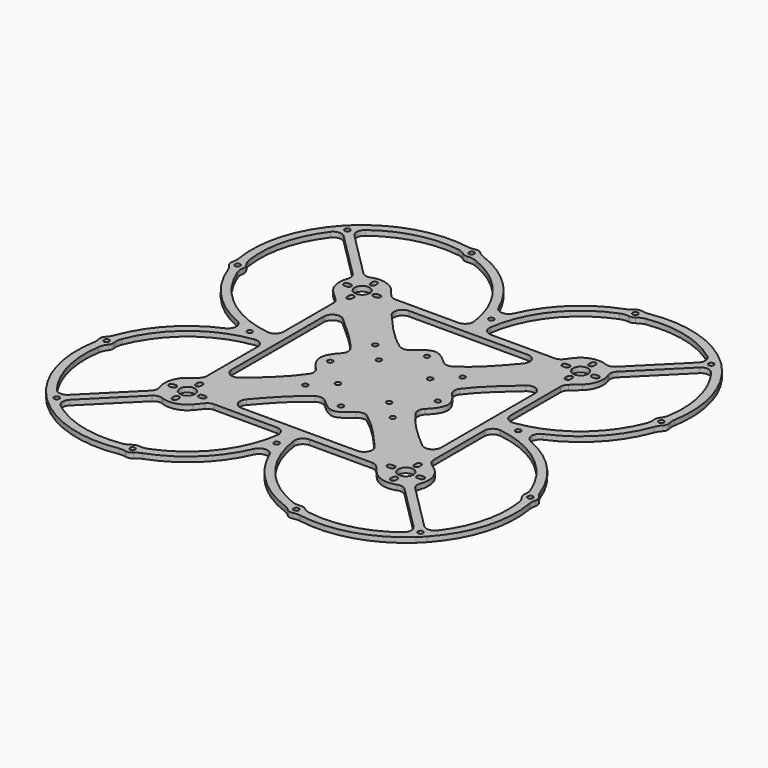
from build123d import *

# Parameters (mm, degrees)
F0_R     = 1.55
F0_R_2   = 4.5
F1_DEPTH = 3


# Not quite as in the source:
# - a feature names something its author has since deleted; it is built from what else it names


with BuildPart() as f1:
    # F0 (on Top) → F1 (new body)
    with BuildSketch(Plane.XY):
        with BuildLine():
            ThreePointArc((4.5936412885, 90.9640892891), (1.5876e-06, 87.9385448385), (-4.5936380583, 90.9640893729))
            ThreePointArc((-4.5936380583, 90.9640893729), (-19.7997665524, 112.7493601662), (-42.3857157583, 126.7386155355))
            ThreePointArc((-42.3857157583, 126.7386155355), (-44.282976849, 127.6715883742), (-45.9416856044, 128.9825892242))
            ThreePointArc((-45.9416856044, 128.9825892242), (-47.711537449, 129.9897804476), (-49.7479021723, 129.9951119953))
            ThreePointArc((-49.7479021723, 129.9951119953), (-51.8387697531, 129.6815665856), (-53.9488258268, 129.814612931))
            ThreePointArc((-53.9488258268, 129.814612931), (-83.7536549239, 128.0187505985), (-109.6908840175, 113.2264179235))
            ThreePointArc((-109.6908840175, 113.2264179235), (-111.492270863, 111.492270863), (-113.2264179235, 109.6908840175))
            ThreePointArc((-113.2264179235, 109.6908840175), (-128.0187505985, 83.7536549239), (-129.814612931, 53.9488258268))
            ThreePointArc((-129.814612931, 53.9488258268), (-129.6815665856, 51.8387697531), (-129.9951119953, 49.7479021723))
            ThreePointArc((-129.9951119953, 49.7479021723), (-129.9897804476, 47.711537449), (-128.9825892242, 45.9416856044))
            ThreePointArc((-128.9825892242, 45.9416856044), (-127.6715883742, 44.282976849), (-126.7386155355, 42.3857157583))
            ThreePointArc((-126.7386155355, 42.3857157583), (-112.7493601662, 19.7997665524), (-90.9640893729, 4.5936380583))
            ThreePointArc((-90.9640893729, 4.5936380583), (-87.9385448385, -1.5876e-06), (-90.9640892891, -4.5936412885))
            ThreePointArc((-90.9640892891, -4.5936412885), (-112.7493564136, -19.7997669532), (-126.7386107311, -42.3857113668))
            ThreePointArc((-126.7386107311, -42.3857113668), (-127.6715848934, -44.2829742089), (-128.9825877652, -45.9416841141))
            ThreePointArc((-128.9825877652, -45.9416841141), (-129.9897804476, -47.711537449), (-129.9951114697, -49.7479041907))
            ThreePointArc((-129.9951114697, -49.7479041907), (-129.6815648767, -51.8387737737), (-129.8146109437, -53.9488320249))
            ThreePointArc((-129.8146109437, -53.9488320249), (-128.0187466409, -83.7536577022), (-113.2264144939, -109.6908833036))
            ThreePointArc((-113.2264144939, -109.6908833036), (-111.4922673823, -111.4922701), (-109.6908804846, -113.2264171062))
            ThreePointArc((-109.6908804846, -113.2264171062), (-83.7536558603, -128.018747189), (-53.9488320249, -129.8146109437))
            ThreePointArc((-53.9488320249, -129.8146109437), (-51.8387737737, -129.6815648767), (-49.7479041907, -129.9951114697))
            ThreePointArc((-49.7479041907, -129.9951114697), (-47.711537449, -129.9897804476), (-45.9416841141, -128.9825877652))
            ThreePointArc((-45.9416841141, -128.9825877652), (-44.2829742089, -127.6715848934), (-42.3857113668, -126.7386107311))
            ThreePointArc((-42.3857113668, -126.7386107311), (-19.7997655576, -112.7493550925), (-4.5936397708, -90.9640857581))
            ThreePointArc((-4.5936397708, -90.9640857581), (0, -87.938541039), (4.5936397708, -90.9640857581))
            ThreePointArc((4.5936397708, -90.9640857581), (19.7997655576, -112.7493550925), (42.3857113668, -126.7386107311))
            ThreePointArc((42.3857113668, -126.7386107311), (44.2829742089, -127.6715848934), (45.9416841141, -128.9825877652))
            ThreePointArc((45.9416841141, -128.9825877652), (47.711537449, -129.9897804476), (49.7479041907, -129.9951114697))
            ThreePointArc((49.7479041907, -129.9951114697), (51.8387737737, -129.6815648767), (53.9488320249, -129.8146109437))
            ThreePointArc((53.9488320249, -129.8146109437), (83.7536567813, -128.0187469149), (109.6908818941, -113.2264158001))
            ThreePointArc((109.6908818941, -113.2264158001), (111.4922687411, -111.4922687411), (113.2264158001, -109.6908818941))
            ThreePointArc((113.2264158001, -109.6908818941), (128.0187469149, -83.7536567813), (129.8146109437, -53.9488320249))
            ThreePointArc((129.8146109437, -53.9488320249), (129.6815648767, -51.8387737737), (129.9951114697, -49.7479041907))
            ThreePointArc((129.9951114697, -49.7479041907), (129.9897804476, -47.711537449), (128.9825877652, -45.9416841141))
            ThreePointArc((128.9825877652, -45.9416841141), (127.6715848934, -44.2829742089), (126.7386107311, -42.3857113668))
            ThreePointArc((126.7386107311, -42.3857113668), (112.7493550925, -19.7997655576), (90.9640857581, -4.5936397708))
            ThreePointArc((90.9640857581, -4.5936397708), (87.938541039, 0), (90.9640857581, 4.5936397708))
            ThreePointArc((90.9640857581, 4.5936397708), (112.7493550925, 19.7997655576), (126.7386107311, 42.3857113668))
            ThreePointArc((126.7386107311, 42.3857113668), (127.6715848934, 44.2829742089), (128.9825877652, 45.9416841141))
            ThreePointArc((128.9825877652, 45.9416841141), (129.9897804476, 47.711537449), (129.9951114697, 49.7479041907))
            ThreePointArc((129.9951114697, 49.7479041907), (129.6815648767, 51.8387737737), (129.8146109437, 53.9488320249))
            ThreePointArc((129.8146109437, 53.9488320249), (128.018747189, 83.7536558603), (113.2264171062, 109.6908804846))
            ThreePointArc((113.2264171062, 109.6908804846), (111.4922701, 111.4922673823), (109.6908833036, 113.2264144939))
            ThreePointArc((109.6908833036, 113.2264144939), (83.7536577022, 128.0187466408), (53.9488320249, 129.8146109437))
            ThreePointArc((53.9488320249, 129.8146109437), (51.8387737737, 129.6815648767), (49.7479041907, 129.9951114697))
            ThreePointArc((49.7479041907, 129.9951114697), (47.711537449, 129.9897804476), (45.9416841141, 128.9825877652))
            ThreePointArc((45.9416841141, 128.9825877652), (44.2829742089, 127.6715848934), (42.3857113668, 126.7386107311))
            ThreePointArc((42.3857113668, 126.7386107311), (19.7997669532, 112.7493564136), (4.5936412885, 90.9640892891))
        make_face()
        with Locations((-108.2905437355, -108.153230011)):
            Circle(F0_R, mode=Mode.SUBTRACT)
        with Locations((-48.7398474892, -126.1242172983)):
            Circle(F0_R, mode=Mode.SUBTRACT)
        with BuildLine():
            Line((-66.5, -74.5), (-66.5, -73))
            ThreePointArc((-66.5, -73), (-65, -71.5), (-63.5, -73))
            Line((-63.5, -73), (-63.5, -74.5))
            ThreePointArc((-63.5, -74.5), (-65, -76), (-66.5, -74.5))
        make_face(mode=Mode.SUBTRACT)
        with Locations((-126.1242172983, -48.7398474892)):
            Circle(F0_R, mode=Mode.SUBTRACT)
        with BuildLine():
            Line((-73, -66.5), (-74.5, -66.5))
            ThreePointArc((-74.5, -66.5), (-76, -65), (-74.5, -63.5))
            Line((-74.5, -63.5), (-73, -63.5))
            ThreePointArc((-73, -63.5), (-71.5, -65), (-73, -66.5))
        make_face(mode=Mode.SUBTRACT)
        with Locations((-79.8885448385, 0)):
            Circle(F0_R, mode=Mode.SUBTRACT)
        with Locations((-65, -65)):
            Circle(F0_R_2, mode=Mode.SUBTRACT)
        with BuildLine():
            ThreePointArc((-57, -66.5), (-58.5, -65), (-57, -63.5))
            Line((-57, -63.5), (-55.5, -63.5))
            ThreePointArc((-55.5, -63.5), (-54, -65), (-55.5, -66.5))
            Line((-55.5, -66.5), (-57, -66.5))
        make_face(mode=Mode.SUBTRACT)
        with BuildLine():
            Line((-66.5, -57), (-66.5, -55.5))
            ThreePointArc((-66.5, -55.5), (-65, -54), (-63.5, -55.5))
            Line((-63.5, -55.5), (-63.5, -57))
            ThreePointArc((-63.5, -57), (-65, -58.5), (-66.5, -57))
        make_face(mode=Mode.SUBTRACT)
        with Locations((48.7398474892, -126.1242172983)):
            Circle(F0_R, mode=Mode.SUBTRACT)
        with Locations((0, -79.8885448385)):
            Circle(F0_R, mode=Mode.SUBTRACT)
        with BuildLine():
            ThreePointArc((66.5, -74.5), (65, -76), (63.5, -74.5))
            Line((63.5, -74.5), (63.5, -73))
            ThreePointArc((63.5, -73), (65, -71.5), (66.5, -73))
            Line((66.5, -73), (66.5, -74.5))
        make_face(mode=Mode.SUBTRACT)
        with Locations((108.2784277556, -108.1560280507)):
            Circle(F0_R, mode=Mode.SUBTRACT)
        with BuildLine():
            ThreePointArc((57, -63.5), (58.5, -65), (57, -66.5))
            Line((57, -66.5), (55.5, -66.5))
            ThreePointArc((55.5, -66.5), (54, -65), (55.5, -63.5))
            Line((55.5, -63.5), (57, -63.5))
        make_face(mode=Mode.SUBTRACT)
        with Locations((65, -65)):
            Circle(F0_R_2, mode=Mode.SUBTRACT)
        with BuildLine():
            ThreePointArc((66.5, -57), (65, -58.5), (63.5, -57))
            Line((63.5, -57), (63.5, -55.5))
            ThreePointArc((63.5, -55.5), (65, -54), (66.5, -55.5))
            Line((66.5, -55.5), (66.5, -57))
        make_face(mode=Mode.SUBTRACT)
        with BuildLine():
            ThreePointArc((-78.7260276961, 75.1904937901), (-77.3700677078, 72.6909557736), (-77.5962746825, 69.8563220777))
            ThreePointArc((-77.5962746825, 69.8563220777), (-78.1774623607, 62.066659629), (-74.3468847944, 55.2590685948))
            ThreePointArc((-74.3468847944, 55.2590685948), (-55.8574100489, 55.0670724866), (-54.5192604238, 73.5090597562))
            ThreePointArc((-54.5192604238, 73.5090597562), (-61.5236729853, 78.0447365051), (-69.8563220777, 77.5962746825))
            ThreePointArc((-69.8563220777, 77.5962746825), (-72.6909557736, 77.3700677078), (-75.1904937901, 78.7260276961))
            Line((-75.1904937901, 78.7260276961), (-102.2950830455, 105.8306169514))
            ThreePointArc((-102.2950830455, 105.8306169514), (-103.7481732445, 109.7032406669), (-101.7873113942, 113.3451778401))
            ThreePointArc((-101.7873113942, 113.3451778401), (-80.0827992563, 123.8478688365), (-56.0022199647, 125.0799671641))
            ThreePointArc((-56.0022199647, 125.0799671641), (-53.4825995412, 124.3550905641), (-51.2379870694, 123.0002296802))
            ThreePointArc((-51.2379870694, 123.0002296802), (-49.7681575294, 122.258654149), (-48.1241365653, 122.1718888632))
            ThreePointArc((-48.1241365653, 122.1718888632), (-45.5030157293, 122.2323762703), (-42.9562600942, 121.6095047758))
            ThreePointArc((-42.9562600942, 121.6095047758), (-17.2773803845, 102.5914096175), (-4.8022395632, 73.1726457399))
            ThreePointArc((-4.8022395632, 73.1726457399), (-5.9909393236, 69.2108685569), (-9.7567877473, 67.5))
            Line((-9.7567877473, 67.5), (-47.2749619701, 67.5))
            ThreePointArc((-47.2749619701, 67.5), (-49.4332948043, 67.989833775), (-51.1687379105, 69.3633602493))
            add(Edge.make_bspline(
                [(-51.1687379105, 69.3633602493), (-47.007111135, 64.1971813129), (-42.9204896878, 59.0857782526), (-38.8861434054, 54.2837422746)],
                knots=[0.0293673697, 0.0293673697, 0.0293673697, 0.0293673697, 0.1393383892, 0.1393383892, 0.1393383892, 0.1393383892], degree=3))
            ThreePointArc((-38.8861434054, 54.2837422746), (-39.5900475875, 59.6117186571), (-35.0578688274, 62.5))
            Line((-35.0578688274, 62.5), (35.6142056633, 62.5))
            ThreePointArc((35.6142056633, 62.5), (40.1396288907, 59.6261572409), (39.4629102085, 54.3082178452))
            add(Edge.make_bspline(
                [(39.4629102085, 54.3082178452), (43.4572386204, 59.1246461501), (47.4477718972, 64.2594353508), (51.4265936274, 69.4628891406)],
                knots=[0.8640600007, 0.8640600007, 0.8640600007, 0.8640600007, 0.9739367654, 0.9739367654, 0.9739367654, 0.9739367654], degree=3))
            ThreePointArc((51.4265936274, 69.4628891406), (49.6699228907, 68.0175032461), (47.4546976535, 67.5))
            Line((47.4546976535, 67.5), (9.7567877473, 67.5))
            ThreePointArc((9.7567877473, 67.5), (5.9909393236, 69.2108685569), (4.8022395632, 73.1726457399))
            ThreePointArc((4.8022395632, 73.1726457399), (17.2773803845, 102.5914096175), (42.9562600942, 121.6095047758))
            ThreePointArc((42.9562600942, 121.6095047758), (45.5030157293, 122.2323762703), (48.1241365653, 122.1718888632))
            ThreePointArc((48.1241365653, 122.1718888632), (49.7681575294, 122.258654149), (51.2379870694, 123.0002296802))
            ThreePointArc((51.2379870694, 123.0002296802), (53.4825995412, 124.3550905641), (56.0022199647, 125.0799671641))
            ThreePointArc((56.0022199647, 125.0799671641), (80.0828001163, 123.8478686161), (101.7873128072, 113.3451767649))
            ThreePointArc((101.7873128072, 113.3451767649), (103.748174551, 109.7032395344), (102.2950842388, 105.8306158614))
            Line((102.2950842388, 105.8306158614), (75.1904941913, 78.7260273982))
            ThreePointArc((75.1904941913, 78.7260273982), (72.6909561352, 77.370067483), (69.8563224458, 77.5962745406))
            ThreePointArc((69.8563224458, 77.5962745406), (61.3181994895, 77.9882387182), (54.2558912586, 73.1739909073))
            ThreePointArc((54.2558912586, 73.1739909073), (55.8750675797, 55.0508488641), (74.0703287451, 55.0010432317))
            ThreePointArc((74.0703287451, 55.0010432317), (78.1350771686, 61.8823489971), (77.5962748245, 69.8563217095))
            ThreePointArc((77.5962748245, 69.8563217095), (77.3700679326, 72.6909554121), (78.7260279939, 75.190493389))
            Line((78.7260279939, 75.190493389), (105.8306180414, 102.2950818521))
            ThreePointArc((105.8306180414, 102.2950818521), (109.7032417994, 103.7481719379), (113.3451789152, 101.7873099812))
            ThreePointArc((113.3451789152, 101.7873099812), (123.8478690569, 80.0827983963), (125.0799671641, 56.0022199647))
            ThreePointArc((125.0799671641, 56.0022199647), (124.3550905641, 53.4825995412), (123.0002296802, 51.2379870694))
            ThreePointArc((123.0002296802, 51.2379870694), (122.258654149, 49.7681575294), (122.1718888632, 48.1241365653))
            ThreePointArc((122.1718888632, 48.1241365653), (122.2323762703, 45.5030157293), (121.6095047758, 42.9562600942))
            ThreePointArc((121.6095047758, 42.9562600942), (102.5914096175, 17.2773803845), (73.1726457399, 4.8022395632))
            ThreePointArc((73.1726457399, 4.8022395632), (69.2108685569, 5.9909393236), (67.5, 9.7567877473))
            Line((67.5, 9.7567877473), (67.5, 46.9024650002))
            ThreePointArc((67.5, 46.9024650002), (67.9450696625, 48.9646506418), (69.2010438482, 50.6597097764))
            add(Edge.make_bspline(
                [(69.2010438482, 50.6597097764), (64.0951140729, 46.1765740091), (59.0182901872, 41.9052788751), (54.2353248312, 37.7820833857)],
                knots=[0.0348728398, 0.0348728398, 0.0348728398, 0.0348728398, 0.1445829675, 0.1445829675, 0.1445829675, 0.1445829675], degree=3))
            ThreePointArc((54.2353248312, 37.7820833857), (59.5828615119, 38.5405267444), (62.5, 33.9950138006))
            Line((62.5, 33.9950138006), (62.5, -35.5495988309))
            ThreePointArc((62.5, -35.5495988309), (59.6206264771, -40.0776164264), (54.2988226622, -39.3904924316))
            add(Edge.make_bspline(
                [(54.2988226622, -39.3904924316), (59.1121784473, -43.4021644694), (64.2467475497, -47.4153572737), (69.4560669959, -51.4128712838)],
                knots=[0.8650150287, 0.8650150287, 0.8650150287, 0.8650150287, 0.9740421792, 0.9740421792, 0.9740421792, 0.9740421792], degree=3))
            ThreePointArc((69.4560669959, -51.4128712838), (68.0156012097, -49.6575734697), (67.5, -47.4462011605))
            Line((67.5, -47.4462011605), (67.5, -9.7567877473))
            ThreePointArc((67.5, -9.7567877473), (69.2108685569, -5.9909393236), (73.1726457399, -4.8022395632))
            ThreePointArc((73.1726457399, -4.8022395632), (102.5914096175, -17.2773803845), (121.6095047758, -42.9562600942))
            ThreePointArc((121.6095047758, -42.9562600942), (122.2323762703, -45.5030157293), (122.1718888632, -48.1241365653))
            ThreePointArc((122.1718888632, -48.1241365653), (122.258654149, -49.7681575294), (123.0002296802, -51.2379870694))
            ThreePointArc((123.0002296802, -51.2379870694), (124.3550905641, -53.4825995412), (125.0799671641, -56.0022199647))
            ThreePointArc((125.0799671641, -56.0022199647), (123.8478688365, -80.0827992563), (113.3451778401, -101.7873113942))
            ThreePointArc((113.3451778401, -101.7873113942), (109.7032406669, -103.7481732445), (105.8306169514, -102.2950830455))
            Line((105.8306169514, -102.2950830455), (78.7260276961, -75.1904937901))
            ThreePointArc((78.7260276961, -75.1904937901), (77.3700677078, -72.6909557736), (77.5962746825, -69.8563220777))
            ThreePointArc((77.5962746825, -69.8563220777), (77.9903375994, -61.3256117442), (73.1862480092, -54.2652273647))
            ThreePointArc((73.1862480092, -54.2652273647), (55.0961710642, -55.8258966427), (54.9219208197, -73.9823337745))
            ThreePointArc((54.9219208197, -73.9823337745), (61.8248103944, -78.1212869403), (69.8563220777, -77.5962746825))
            ThreePointArc((69.8563220777, -77.5962746825), (72.6909557736, -77.3700677078), (75.1904937901, -78.7260276961))
            Line((75.1904937901, -78.7260276961), (102.2950830455, -105.8306169514))
            ThreePointArc((102.2950830455, -105.8306169514), (103.7481732445, -109.7032406669), (101.7873113942, -113.3451778401))
            ThreePointArc((101.7873113942, -113.3451778401), (80.0827992563, -123.8478688365), (56.0022199647, -125.0799671641))
            ThreePointArc((56.0022199647, -125.0799671641), (53.4825995412, -124.3550905641), (51.2379870694, -123.0002296802))
            ThreePointArc((51.2379870694, -123.0002296802), (49.7681575294, -122.258654149), (48.1241365653, -122.1718888632))
            ThreePointArc((48.1241365653, -122.1718888632), (45.5030157293, -122.2323762703), (42.9562600942, -121.6095047758))
            ThreePointArc((42.9562600942, -121.6095047758), (17.2773803845, -102.5914096175), (4.8022395632, -73.1726457399))
            ThreePointArc((4.8022395632, -73.1726457399), (5.9909393236, -69.2108685569), (9.7567877473, -67.5))
            Line((9.7567877473, -67.5), (46.9610754937, -67.5))
            ThreePointArc((46.9610754937, -67.5), (49.0351777215, -67.9504835478), (50.7355403773, -69.2207600206))
            add(Edge.make_bspline(
                [(50.7355403773, -69.2207600206), (46.2776004608, -64.0895900624), (42.0082462932, -59.0081310929), (37.8793761718, -54.2306155101)],
                knots=[0.0336445481, 0.0336445481, 0.0336445481, 0.0336445481, 0.1425668185, 0.1425668185, 0.1425668185, 0.1425668185], degree=3))
            ThreePointArc((37.8793761718, -54.2306155101), (38.6431792121, -59.5800333592), (34.0963714061, -62.5))
            Line((34.0963714061, -62.5), (-34.6716965747, -62.5))
            ThreePointArc((-34.6716965747, -62.5), (-39.2116462302, -59.594959934), (-38.4761016269, -54.25554285))
            add(Edge.make_bspline(
                [(-38.4761016269, -54.25554285), (-42.5524815665, -59.0354489236), (-46.7247402937, -64.1334390375), (-51.0163929038, -69.3081210856)],
                knots=[0.86152407, 0.86152407, 0.86152407, 0.86152407, 0.9696650908, 0.9696650908, 0.9696650908, 0.9696650908], degree=3))
            ThreePointArc((-51.0163929038, -69.3081210856), (-49.2938689584, -67.974550046), (-47.1677686047, -67.5))
            Line((-47.1677686047, -67.5), (-9.7567877474, -67.5))
            ThreePointArc((-9.7567877474, -67.5), (-5.9909393237, -69.2108685569), (-4.8022395633, -73.1726457399))
            ThreePointArc((-4.8022395633, -73.1726457399), (-17.2773803846, -102.5914096175), (-42.9562600944, -121.6095047758))
            ThreePointArc((-42.9562600944, -121.6095047758), (-45.5030157294, -122.2323762703), (-48.1241365654, -122.1718888632))
            ThreePointArc((-48.1241365654, -122.1718888632), (-49.7681575294, -122.258654149), (-51.2379870693, -123.0002296802))
            ThreePointArc((-51.2379870693, -123.0002296802), (-53.4825995411, -124.355090564), (-56.0022199645, -125.079967164))
            ThreePointArc((-56.0022199645, -125.079967164), (-80.0827983962, -123.8478690568), (-101.7873099811, -113.3451789152))
            ThreePointArc((-101.7873099811, -113.3451789152), (-103.7481719378, -109.7032417994), (-102.295081852, -105.8306180414))
            Line((-102.295081852, -105.8306180414), (-75.190493389, -78.7260279939))
            ThreePointArc((-75.190493389, -78.7260279939), (-72.6909554121, -77.3700679326), (-69.8563217095, -77.5962748245))
            ThreePointArc((-69.8563217095, -77.5962748245), (-61.6280970797, -78.0721180647), (-54.6566830252, -73.6755860873))
            ThreePointArc((-54.6566830252, -73.6755860873), (-55.3115936341, -55.5986818962), (-73.3606290294, -54.4004772639))
            ThreePointArc((-73.3606290294, -54.4004772639), (-78.019936228, -61.431910789), (-77.5962745406, -69.8563224458))
            ThreePointArc((-77.5962745406, -69.8563224458), (-77.370067483, -72.6909561352), (-78.7260273982, -75.1904941913))
            Line((-78.7260273982, -75.1904941913), (-105.8306158613, -102.2950842388))
            ThreePointArc((-105.8306158613, -102.2950842388), (-109.7032395344, -103.7481745509), (-113.3451767648, -101.7873128071))
            ThreePointArc((-113.3451767648, -101.7873128071), (-123.847868616, -80.0828001162), (-125.079967164, -56.0022199645))
            ThreePointArc((-125.079967164, -56.0022199645), (-124.355090564, -53.4825995411), (-123.0002296802, -51.2379870693))
            ThreePointArc((-123.0002296802, -51.2379870693), (-122.258654149, -49.7681575294), (-122.1718888632, -48.1241365654))
            ThreePointArc((-122.1718888632, -48.1241365654), (-122.2323762703, -45.5030157294), (-121.6095047758, -42.9562600944))
            ThreePointArc((-121.6095047758, -42.9562600944), (-102.5915462524, -17.277488013), (-73.1729904451, -4.8022863626))
            ThreePointArc((-73.1729904451, -4.8022863626), (-69.2111956733, -5.9909728541), (-67.5003163344, -9.7568306947))
            Line((-67.5003163344, -9.7568306947), (-67.5003163328, -47.353236691))
            ThreePointArc((-67.5003163328, -47.353236691), (-68.0006204029, -49.5333138774), (-69.4014109482, -51.2771104681))
            add(Edge.make_bspline(
                [(-54.2790618736, -39.0485616103), (-59.0828616964, -43.094423634), (-64.2057413604, -47.1737958924), (-69.4014109482, -51.2771104681)],
                knots=[0.8641405018, 0.8641405018, 0.8641405018, 0.8641405018, 0.9725362801, 0.9725362801, 0.9725362801, 0.9725362801], degree=3))
            ThreePointArc((-54.2790618736, -39.0485616103), (-59.6089463445, -39.7576935316), (-62.5, -35.2242240748))
            Line((-62.5, -35.2242240748), (-62.5, 33.4095018987))
            ThreePointArc((-62.5, 33.4095018987), (-59.5674116994, 37.9620625919), (-54.209676454, 37.1743087945))
            add(Edge.make_bspline(
                [(-69.1233391423, 50.3680202269), (-64.0476785875, 45.7195000527), (-58.9859996351, 41.3486659558), (-54.209676454, 37.1743087945)],
                knots=[0.0376140132, 0.0376140132, 0.0376140132, 0.0376140132, 0.147134592, 0.147134592, 0.147134592, 0.147134592], degree=3))
            ThreePointArc((-69.1233391423, 50.3680202269), (-67.9240249358, 48.6950792761), (-67.5003163367, 46.6807414163))
            Line((-67.5003163367, 46.6807414163), (-67.5003163352, 9.7568306951))
            ThreePointArc((-67.5003163352, 9.7568306951), (-69.211195674, 5.9909728542), (-73.1729904459, 4.8022863626))
            ThreePointArc((-73.1729904459, 4.8022863626), (-102.5915462527, 17.2774880132), (-121.6095047758, 42.9562600942))
            ThreePointArc((-121.6095047758, 42.9562600942), (-122.2323762703, 45.5030157293), (-122.1718888632, 48.1241365653))
            ThreePointArc((-122.1718888632, 48.1241365653), (-122.258654149, 49.7681575294), (-123.0002296802, 51.2379870694))
            ThreePointArc((-123.0002296802, 51.2379870694), (-124.3550905641, 53.4825995412), (-125.0799671641, 56.0022199647))
            ThreePointArc((-125.0799671641, 56.0022199647), (-123.8478688365, 80.0827992563), (-113.3451778401, 101.7873113942))
            ThreePointArc((-113.3451778401, 101.7873113942), (-109.7032406669, 103.7481732445), (-105.8306169514, 102.2950830455))
            Line((-105.8306169514, 102.2950830455), (-78.7260276961, 75.1904937901))
        make_face(mode=Mode.SUBTRACT)
        with BuildLine():
            ThreePointArc((74.5, -63.5), (76, -65), (74.5, -66.5))
            Line((74.5, -66.5), (73, -66.5))
            ThreePointArc((73, -66.5), (71.5, -65), (73, -63.5))
            Line((73, -63.5), (74.5, -63.5))
        make_face(mode=Mode.SUBTRACT)
        with Locations((126.1242172983, -48.7398474892)):
            Circle(F0_R, mode=Mode.SUBTRACT)
        with Locations((79.8885448385, 0)):
            Circle(F0_R, mode=Mode.SUBTRACT)
        with Locations((-126.1242172983, 48.7398474892)):
            Circle(F0_R, mode=Mode.SUBTRACT)
        with BuildLine():
            ThreePointArc((-73, 66.5), (-71.5, 65), (-73, 63.5))
            Line((-73, 63.5), (-74.5, 63.5))
            ThreePointArc((-74.5, 63.5), (-76, 65), (-74.5, 66.5))
            Line((-74.5, 66.5), (-73, 66.5))
        make_face(mode=Mode.SUBTRACT)
        with BuildLine():
            ThreePointArc((-63.5, 55.5), (-65, 54), (-66.5, 55.5))
            Line((-66.5, 55.5), (-66.5, 57))
            ThreePointArc((-66.5, 57), (-65, 58.5), (-63.5, 57))
            Line((-63.5, 57), (-63.5, 55.5))
        make_face(mode=Mode.SUBTRACT)
        with Locations((-65, 65)):
            Circle(F0_R_2, mode=Mode.SUBTRACT)
        with BuildLine():
            Line((-55.5, 63.5), (-57, 63.5))
            ThreePointArc((-57, 63.5), (-58.5, 65), (-57, 66.5))
            Line((-57, 66.5), (-55.5, 66.5))
            ThreePointArc((-55.5, 66.5), (-54, 65), (-55.5, 63.5))
        make_face(mode=Mode.SUBTRACT)
        with Locations((-108.3014905595, 108.1507019099)):
            Circle(F0_R, mode=Mode.SUBTRACT)
        with BuildLine():
            ThreePointArc((-63.5, 73), (-65, 71.5), (-66.5, 73))
            Line((-66.5, 73), (-66.5, 74.5))
            ThreePointArc((-66.5, 74.5), (-65, 76), (-63.5, 74.5))
            Line((-63.5, 74.5), (-63.5, 73))
        make_face(mode=Mode.SUBTRACT)
        with Locations((-48.7398474892, 126.1242172983)):
            Circle(F0_R, mode=Mode.SUBTRACT)
        with BuildLine():
            Line((63.5, 55.5), (63.5, 57))
            ThreePointArc((63.5, 57), (65, 58.5), (66.5, 57))
            Line((66.5, 57), (66.5, 55.5))
            ThreePointArc((66.5, 55.5), (65, 54), (63.5, 55.5))
        make_face(mode=Mode.SUBTRACT)
        with BuildLine():
            Line((55.5, 66.5), (57, 66.5))
            ThreePointArc((57, 66.5), (58.5, 65), (57, 63.5))
            Line((57, 63.5), (55.5, 63.5))
            ThreePointArc((55.5, 63.5), (54, 65), (55.5, 66.5))
        make_face(mode=Mode.SUBTRACT)
        with Locations((65, 65)):
            Circle(F0_R_2, mode=Mode.SUBTRACT)
        with BuildLine():
            Line((74.5, 63.5), (73, 63.5))
            ThreePointArc((73, 63.5), (71.5, 65), (73, 66.5))
            Line((73, 66.5), (74.5, 66.5))
            ThreePointArc((74.5, 66.5), (76, 65), (74.5, 63.5))
        make_face(mode=Mode.SUBTRACT)
        with Locations((126.1242172983, 48.7398474892)):
            Circle(F0_R, mode=Mode.SUBTRACT)
        with Locations((0, 79.8885448385)):
            Circle(F0_R, mode=Mode.SUBTRACT)
        with BuildLine():
            Line((66.5, 74.5), (66.5, 73))
            ThreePointArc((66.5, 73), (65, 71.5), (63.5, 73))
            Line((63.5, 73), (63.5, 74.5))
            ThreePointArc((63.5, 74.5), (65, 76), (66.5, 74.5))
        make_face(mode=Mode.SUBTRACT)
        with Locations((48.7398474892, 126.1242172983)):
            Circle(F0_R, mode=Mode.SUBTRACT)
        with Locations((108.153230011, 108.2905437356)):
            Circle(F0_R, mode=Mode.SUBTRACT)
        with BuildLine():
            ThreePointArc((-54.5192604238, 73.5090597562), (-55.8574100489, 55.0670724866), (-74.3468847944, 55.2590685948))
            add(Edge.make_bspline(
                [(-74.3468847944, 55.2590685948), (-72.6113826473, 53.5937721304), (-70.8665363109, 51.9645192675), (-69.1233391423, 50.3680202269)],
                knots=[0, 0, 0, 0, 0.0376140132, 0.0376140132, 0.0376140132, 0.0376140132], degree=3))
            add(Edge.make_bspline(
                [(-69.1233391423, 50.3680202269), (-64.0476785875, 45.7195000527), (-58.9859996351, 41.3486659558), (-54.209676454, 37.1743087945)],
                knots=[0.0376140132, 0.0376140132, 0.0376140132, 0.0376140132, 0.147134592, 0.147134592, 0.147134592, 0.147134592], degree=3))
            add(Edge.make_bspline(
                [(-54.209676454, 37.1743087945), (-45.5797737114, 29.6320435523), (-37.8814314438, 22.7311886683), (-32.7153317801, 15.99273753)],
                knots=[0.147134592, 0.147134592, 0.147134592, 0.147134592, 0.3450173373, 0.3450173373, 0.3450173373, 0.3450173373], degree=3))
            add(Edge.make_bspline(
                [(-32.7153317801, 15.99273753), (-31.7544055806, 14.7393443196), (-30.8810906196, 13.4915699994), (-30.1056880744, 12.2463319262)],
                knots=[0.3450173373, 0.3450173373, 0.3450173373, 0.3450173373, 0.3818247408, 0.3818247408, 0.3818247408, 0.3818247408], degree=3))
            add(Edge.make_bspline(
                [(-30.1056880744, 12.2463319262), (-27.5692779158, 8.1730482903), (-24.5965263706, 0.0936378541), (-27.2387091268, -8.3077722195), (-29.6226546248, -12.5690364936)],
                knots=[0.3818247408, 0.3818247408, 0.3818247408, 0.3818247408, 0.5022250058, 0.622241972, 0.622241972, 0.622241972, 0.622241972], degree=3))
            add(Edge.make_bspline(
                [(-29.6226546248, -12.5690364936), (-30.3158734916, -13.8081540799), (-31.099141907, -15.0529586505), (-31.9642401019, -16.3031308824)],
                knots=[0.622241972, 0.622241972, 0.622241972, 0.622241972, 0.6571412704, 0.6571412704, 0.6571412704, 0.6571412704], degree=3))
            add(Edge.make_bspline(
                [(-31.9642401019, -16.3031308824), (-37.0954223742, -23.718314074), (-45.105430893, -31.3223351702), (-54.2790618736, -39.0485616103)],
                knots=[0.6571412704, 0.6571412704, 0.6571412704, 0.6571412704, 0.8641405018, 0.8641405018, 0.8641405018, 0.8641405018], degree=3))
            add(Edge.make_bspline(
                [(-54.2790618736, -39.0485616103), (-59.0828616964, -43.094423634), (-64.2057413604, -47.1737958924), (-69.4014109482, -51.2771104681)],
                knots=[0.8641405018, 0.8641405018, 0.8641405018, 0.8641405018, 0.9725362801, 0.9725362801, 0.9725362801, 0.9725362801], degree=3))
            add(Edge.make_bspline(
                [(-69.4014109482, -51.2771104681), (-70.7178128987, -52.3167476543), (-72.0388875207, -53.3579217921), (-73.3606290294, -54.4004772639)],
                knots=[0.9725362801, 0.9725362801, 0.9725362801, 0.9725362801, 1, 1, 1, 1], degree=3))
            ThreePointArc((-73.3606290294, -54.4004772639), (-55.3115936341, -55.5986818962), (-54.6566830252, -73.6755860873))
            add(Edge.make_bspline(
                [(-51.0163929038, -69.3081210856), (-52.2202551514, -70.7596841376), (-53.4335121775, -72.2172818685), (-54.6566830252, -73.6755860873)],
                knots=[0.9696650908, 0.9696650908, 0.9696650908, 0.9696650908, 1, 1, 1, 1], degree=3))
            add(Edge.make_bspline(
                [(-38.4761016269, -54.25554285), (-42.5524815665, -59.0354489236), (-46.7247402937, -64.1334390375), (-51.0163929038, -69.3081210856)],
                knots=[0.86152407, 0.86152407, 0.86152407, 0.86152407, 0.9696650908, 0.9696650908, 0.9696650908, 0.9696650908], degree=3))
            add(Edge.make_bspline(
                [(-15.7360450393, -31.8416919699), (-23.0709377017, -36.9605236646), (-30.5942962957, -45.0134482139), (-38.4761016269, -54.25554285)],
                knots=[0.6524300978, 0.6524300978, 0.6524300978, 0.6524300978, 0.86152407, 0.86152407, 0.86152407, 0.86152407], degree=3))
            add(Edge.make_bspline(
                [(-12.477120742, -29.7592614372), (-13.5596368679, -30.3847557024), (-14.6457588788, -31.0808094851), (-15.7360450393, -31.8416919699)],
                knots=[0.6213495797, 0.6213495797, 0.6213495797, 0.6213495797, 0.6524300978, 0.6524300978, 0.6524300978, 0.6524300978], degree=3))
            add(Edge.make_bspline(
                [(12.3175276915, -29.9149197418), (8.1902094221, -27.4521418277), (0.0009395531, -24.6081106332), (-8.2746234397, -27.3309946433), (-12.477120742, -29.7592614372)],
                knots=[0.3806340257, 0.3806340257, 0.3806340257, 0.3806340257, 0.500690136, 0.6213495797, 0.6213495797, 0.6213495797, 0.6213495797], degree=3))
            add(Edge.make_bspline(
                [(15.5878401798, -32.071279466), (14.4939747649, -31.2842343393), (13.4042625324, -30.5633762915), (12.3175276915, -29.9149197418)],
                knots=[0.3490229046, 0.3490229046, 0.3490229046, 0.3490229046, 0.3806340257, 0.3806340257, 0.3806340257, 0.3806340257], degree=3))
            add(Edge.make_bspline(
                [(37.8793761718, -54.2306155101), (30.0533332369, -45.1751012959), (22.7320085602, -37.2115671391), (15.5878401798, -32.071279466)],
                knots=[0.1425668185, 0.1425668185, 0.1425668185, 0.1425668185, 0.3490229046, 0.3490229046, 0.3490229046, 0.3490229046], degree=3))
            add(Edge.make_bspline(
                [(50.7355403773, -69.2207600206), (46.2776004608, -64.0895900624), (42.0082462932, -59.0081310929), (37.8793761718, -54.2306155101)],
                knots=[0.0336445481, 0.0336445481, 0.0336445481, 0.0336445481, 0.1425668185, 0.1425668185, 0.1425668185, 0.1425668185], degree=3))
            add(Edge.make_bspline(
                [(54.9219208197, -73.9823337745), (53.5075225493, -72.3953945536), (52.112534936, -70.8057058127), (50.7355403773, -69.2207600206)],
                knots=[0, 0, 0, 0, 0.0336445481, 0.0336445481, 0.0336445481, 0.0336445481], degree=3))
            ThreePointArc((54.9219208197, -73.9823337745), (55.0961710642, -55.8258966427), (73.1862480092, -54.2652273647))
            add(Edge.make_bspline(
                [(69.4560669959, -51.4128712838), (70.6963321973, -52.3646227688), (71.940834612, -53.3154855034), (73.1862480092, -54.2652273647)],
                knots=[0.9740421792, 0.9740421792, 0.9740421792, 0.9740421792, 1, 1, 1, 1], degree=3))
            add(Edge.make_bspline(
                [(54.2988226622, -39.3904924316), (59.1121784473, -43.4021644694), (64.2467475497, -47.4153572737), (69.4560669959, -51.4128712838)],
                knots=[0.8650150287, 0.8650150287, 0.8650150287, 0.8650150287, 0.9740421792, 0.9740421792, 0.9740421792, 0.9740421792], degree=3))
            add(Edge.make_bspline(
                [(31.7459765479, -16.2369208779), (36.8685062051, -23.8659236611), (44.9819221427, -31.6253591313), (54.2988226622, -39.3904924316)],
                knots=[0.6539782468, 0.6539782468, 0.6539782468, 0.6539782468, 0.8650150287, 0.8650150287, 0.8650150287, 0.8650150287], degree=3))
            add(Edge.make_bspline(
                [(29.5219284636, -12.5813755873), (30.1816388577, -13.7962022099), (30.9254369782, -15.0148881949), (31.7459765479, -16.2369208779)],
                knots=[0.620173849, 0.620173849, 0.620173849, 0.620173849, 0.6539782468, 0.6539782468, 0.6539782468, 0.6539782468], degree=3))
            add(Edge.make_bspline(
                [(29.9400645414, 12.3562593878), (27.4904286095, 8.253307767), (24.6482914319, 0.0993554776), (27.2148947835, -8.3330782148), (29.5219284636, -12.5813755873)],
                knots=[0.3828924385, 0.3828924385, 0.3828924385, 0.3828924385, 0.5019585155, 0.620173849, 0.620173849, 0.620173849, 0.620173849], degree=3))
            add(Edge.make_bspline(
                [(32.387471575, 16.0209488062), (31.487130896, 14.7969542017), (30.668363937, 13.5761048132), (29.9400645414, 12.3562593878)],
                knots=[0.3474929937, 0.3474929937, 0.3474929937, 0.3474929937, 0.3828924385, 0.3828924385, 0.3828924385, 0.3828924385], degree=3))
            add(Edge.make_bspline(
                [(54.2353248312, 37.7820833857), (45.3891804875, 30.1561902961), (37.5482347411, 23.0369000102), (32.387471575, 16.0209488062)],
                knots=[0.1445829675, 0.1445829675, 0.1445829675, 0.1445829675, 0.3474929937, 0.3474929937, 0.3474929937, 0.3474929937], degree=3))
            add(Edge.make_bspline(
                [(69.2010438482, 50.6597097764), (64.0951140729, 46.1765740091), (59.0182901872, 41.9052788751), (54.2353248312, 37.7820833857)],
                knots=[0.0348728398, 0.0348728398, 0.0348728398, 0.0348728398, 0.1445829675, 0.1445829675, 0.1445829675, 0.1445829675], degree=3))
            add(Edge.make_bspline(
                [(74.0703287451, 55.0010432317), (72.4499615375, 53.5311635631), (70.8240323045, 52.0847347804), (69.2010438482, 50.6597097764)],
                knots=[0, 0, 0, 0, 0.0348728398, 0.0348728398, 0.0348728398, 0.0348728398], degree=3))
            ThreePointArc((74.0703287451, 55.0010432317), (55.8750675797, 55.0508488641), (54.2558912586, 73.1739909073))
            add(Edge.make_bspline(
                [(51.4265936274, 69.4628891406), (52.3703870168, 70.6971704484), (53.3135214459, 71.9353152278), (54.2558912586, 73.1739909073)],
                knots=[0.9739367654, 0.9739367654, 0.9739367654, 0.9739367654, 1, 1, 1, 1], degree=3))
            add(Edge.make_bspline(
                [(39.4629102085, 54.3082178452), (43.4572386204, 59.1246461501), (47.4477718972, 64.2594353508), (51.4265936274, 69.4628891406)],
                knots=[0.8640600007, 0.8640600007, 0.8640600007, 0.8640600007, 0.9739367654, 0.9739367654, 0.9739367654, 0.9739367654], degree=3))
            add(Edge.make_bspline(
                [(16.0277732624, 31.5601593801), (23.8144639959, 36.6758763345), (31.6459546013, 44.8824014468), (39.4629102085, 54.3082178452)],
                knots=[0.6490296618, 0.6490296618, 0.6490296618, 0.6490296618, 0.8640600007, 0.8640600007, 0.8640600007, 0.8640600007], degree=3))
            add(Edge.make_bspline(
                [(12.63212765, 29.5293297846), (13.7629393959, 30.1370057165), (14.8948821775, 30.8158701398), (16.0277732624, 31.5601593801)],
                knots=[0.6177447473, 0.6177447473, 0.6177447473, 0.6177447473, 0.6490296618, 0.6490296618, 0.6490296618, 0.6490296618], degree=3))
            add(Edge.make_bspline(
                [(-12.5423950306, 29.6621706825), (-8.3687174631, 27.3442678436), (-0.0340331605, 24.699772843), (8.4024067679, 27.2563611954), (12.63212765, 29.5293297846)],
                knots=[0.3834666456, 0.3834666456, 0.3834666456, 0.3834666456, 0.5007257504, 0.6177447473, 0.6177447473, 0.6177447473, 0.6177447473], degree=3))
            add(Edge.make_bspline(
                [(-15.948348592, 31.7675257886), (-14.8125086537, 30.9963498788), (-13.6773755118, 30.292495962), (-12.5423950306, 29.6621706825)],
                knots=[0.3515794687, 0.3515794687, 0.3515794687, 0.3515794687, 0.3834666456, 0.3834666456, 0.3834666456, 0.3834666456], degree=3))
            add(Edge.make_bspline(
                [(-38.8861434054, 54.2837422746), (-31.0999647029, 45.0159433197), (-23.5085002785, 36.9004733616), (-15.948348592, 31.7675257886)],
                knots=[0.1393383892, 0.1393383892, 0.1393383892, 0.1393383892, 0.3515794687, 0.3515794687, 0.3515794687, 0.3515794687], degree=3))
            add(Edge.make_bspline(
                [(-51.1687379105, 69.3633602493), (-47.007111135, 64.1971813129), (-42.9204896878, 59.0857782526), (-38.8861434054, 54.2837422746)],
                knots=[0.0293673697, 0.0293673697, 0.0293673697, 0.0293673697, 0.1393383892, 0.1393383892, 0.1393383892, 0.1393383892], degree=3))
            add(Edge.make_bspline(
                [(-54.5192604238, 73.5090597562), (-53.3967820872, 72.126485951), (-52.2800855412, 70.7429699621), (-51.1687379105, 69.3633602493)],
                knots=[0, 0, 0, 0, 0.0293673697, 0.0293673697, 0.0293673697, 0.0293673697], degree=3))
        make_face()
        with Locations((-26, -26)):
            Circle(F0_R, mode=Mode.SUBTRACT)
        with Locations((-15.25, -15.25)):
            Circle(F0_R, mode=Mode.SUBTRACT)
        with Locations((26, -26)):
            Circle(F0_R, mode=Mode.SUBTRACT)
        with Locations((15.25, -15.25)):
            Circle(F0_R, mode=Mode.SUBTRACT)
        with Locations((-15.25, 15.25)):
            Circle(F0_R, mode=Mode.SUBTRACT)
        with Locations((-26, 26)):
            Circle(F0_R, mode=Mode.SUBTRACT)
        with Locations((15.25, 15.25)):
            Circle(F0_R, mode=Mode.SUBTRACT)
        with Locations((26, 26)):
            Circle(F0_R, mode=Mode.SUBTRACT)
        with BuildLine():
            add(Edge.make_bspline(
                [(-30.1056880744, 12.2463319262), (-27.5692779158, 8.1730482903), (-24.5965263706, 0.0936378541), (-27.2387091268, -8.3077722195), (-29.6226546248, -12.5690364936)],
                knots=[0.3818247408, 0.3818247408, 0.3818247408, 0.3818247408, 0.5022250058, 0.622241972, 0.622241972, 0.622241972, 0.622241972], degree=3))
            add(Edge.make_bspline(
                [(-30.1056880744, 12.2463319262), (-31.1933936255, 11.3200095766), (-32.1965910555, 10.3935165414), (-33.0970226063, 9.4666244852)],
                knots=[0, 0, 0, 0, 0.1127085337, 0.1127085337, 0.1127085337, 0.1127085337], degree=3))
            add(Edge.make_bspline(
                [(-33.0970226063, 9.4666244852), (-36.1551134785, 6.318667115), (-39.9750656625, -0.1118316712), (-35.8873186561, -6.5986964156), (-32.5526714682, -9.9101121862)],
                knots=[0.1127085337, 0.1127085337, 0.1127085337, 0.1127085337, 0.4954949184, 0.8935049255, 0.8935049255, 0.8935049255, 0.8935049255], degree=3))
            add(Edge.make_bspline(
                [(-32.5526714682, -9.9101121862), (-31.6604238004, -10.7961438507), (-30.6786186891, -11.6825151808), (-29.6226546248, -12.5690364936)],
                knots=[0.8935049255, 0.8935049255, 0.8935049255, 0.8935049255, 1, 1, 1, 1], degree=3))
        make_face()
        with Locations((-32.05, 0)):
            Circle(F0_R, mode=Mode.SUBTRACT)
        with BuildLine():
            add(Edge.make_bspline(
                [(29.9400645414, 12.3562593878), (30.9576341295, 11.4337447532), (31.9257783104, 10.511183949), (32.8151259954, 9.5884517113)],
                knots=[0, 0, 0, 0, 0.1113309647, 0.1113309647, 0.1113309647, 0.1113309647], degree=3))
            add(Edge.make_bspline(
                [(29.9400645414, 12.3562593878), (27.4904286095, 8.253307767), (24.6482914319, 0.0993554776), (27.2148947835, -8.3330782148), (29.5219284636, -12.5813755873)],
                knots=[0.3828924385, 0.3828924385, 0.3828924385, 0.3828924385, 0.5019585155, 0.620173849, 0.620173849, 0.620173849, 0.620173849], degree=3))
            add(Edge.make_bspline(
                [(32.3538903894, -9.9217654649), (31.4712777739, -10.8081887947), (30.5188378125, -11.6947614064), (29.5219284636, -12.5813755873)],
                knots=[0.8936751921, 0.8936751921, 0.8936751921, 0.8936751921, 1, 1, 1, 1], degree=3))
            add(Edge.make_bspline(
                [(32.8151259954, 9.5884517113), (35.8919952294, 6.3960822007), (40.2259188659, -0.0923036316), (35.6508652368, -6.6105558007), (32.3538903894, -9.9217654649)],
                knots=[0.1113309647, 0.1113309647, 0.1113309647, 0.1113309647, 0.4965018329, 0.8936751921, 0.8936751921, 0.8936751921, 0.8936751921], degree=3))
        make_face()
        with Locations((32.05, 0)):
            Circle(F0_R, mode=Mode.SUBTRACT)
        with BuildLine():
            add(Edge.make_bspline(
                [(-9.7504172108, 32.2282803425), (-10.6811163485, 31.3701306913), (-11.6117483022, 30.4945574622), (-12.5423950306, 29.6621706825)],
                knots=[0.8889148955, 0.8889148955, 0.8889148955, 0.8889148955, 1, 1, 1, 1], degree=3))
            add(Edge.make_bspline(
                [(-12.5423950306, 29.6621706825), (-8.3687174631, 27.3442678436), (-0.0340331605, 24.699772843), (8.4024067679, 27.2563611954), (12.63212765, 29.5293297846)],
                knots=[0.3834666456, 0.3834666456, 0.3834666456, 0.3834666456, 0.5007257504, 0.6177447473, 0.6177447473, 0.6177447473, 0.6177447473], degree=3))
            add(Edge.make_bspline(
                [(12.63212765, 29.5293297846), (11.7146579557, 30.3555633147), (10.7971740578, 31.2232958312), (9.8797533225, 32.0753469391)],
                knots=[0, 0, 0, 0, 0.1091548671, 0.1091548671, 0.1091548671, 0.1091548671], degree=3))
            add(Edge.make_bspline(
                [(9.8797533225, 32.0753469391), (6.5844922479, 35.1358084494), (0.032415079, 40.8201623203), (-6.5022577903, 35.2232405405), (-9.7504172108, 32.2282803425)],
                knots=[0.1091548671, 0.1091548671, 0.1091548671, 0.1091548671, 0.5012255615, 0.8889148955, 0.8889148955, 0.8889148955, 0.8889148955], degree=3))
        make_face()
        with Locations((0, 32.05)):
            Circle(F0_R, mode=Mode.SUBTRACT)
        with BuildLine():
            add(Edge.make_bspline(
                [(12.3175276915, -29.9149197418), (8.1902094221, -27.4521418277), (0.0009395531, -24.6081106332), (-8.2746234397, -27.3309946433), (-12.477120742, -29.7592614372)],
                knots=[0.3806340257, 0.3806340257, 0.3806340257, 0.3806340257, 0.500690136, 0.6213495797, 0.6213495797, 0.6213495797, 0.6213495797], degree=3))
            add(Edge.make_bspline(
                [(-9.5662074569, -32.1929920889), (-10.536440028, -31.336779913), (-11.5068279854, -30.4960757428), (-12.477120742, -29.7592614372)],
                knots=[0.8830576196, 0.8830576196, 0.8830576196, 0.8830576196, 1, 1, 1, 1], degree=3))
            add(Edge.make_bspline(
                [(9.364510034, -32.3763138394), (6.2475661392, -35.1191976173), (-0.0417323846, -40.9343557665), (-6.3728100162, -35.0111058616), (-9.5662074569, -32.1929920889)],
                knots=[0.1195687557, 0.1195687557, 0.1195687557, 0.1195687557, 0.4981566076, 0.8830576196, 0.8830576196, 0.8830576196, 0.8830576196], degree=3))
            add(Edge.make_bspline(
                [(12.3175276915, -29.9149197418), (11.3331783351, -30.6577830151), (10.3489291093, -31.5100335329), (9.364510034, -32.3763138394)],
                knots=[0, 0, 0, 0, 0.1195687557, 0.1195687557, 0.1195687557, 0.1195687557], degree=3))
        make_face()
        with Locations((0, -32.05)):
            Circle(F0_R, mode=Mode.SUBTRACT)
        with BuildLine():
            add(Edge.make_bspline(
                [(-32.7153317801, 15.99273753), (-31.7544055806, 14.7393443196), (-30.8810906196, 13.4915699994), (-30.1056880744, 12.2463319262)],
                knots=[0.3450173373, 0.3450173373, 0.3450173373, 0.3450173373, 0.3818247408, 0.3818247408, 0.3818247408, 0.3818247408], degree=3))
            ThreePointArc((-32.7153317801, 15.99273753), (-31.6919065838, 12.6586623249), (-33.0970226063, 9.4666244852))
            add(Edge.make_bspline(
                [(-30.1056880744, 12.2463319262), (-31.1933936255, 11.3200095766), (-32.1965910555, 10.3935165414), (-33.0970226063, 9.4666244852)],
                knots=[0, 0, 0, 0, 0.1127085337, 0.1127085337, 0.1127085337, 0.1127085337], degree=3))
        make_face()
        with BuildLine():
            ThreePointArc((32.8151259954, 9.5884517113), (31.4261989254, 12.7265755986), (32.387471575, 16.0209488062))
            add(Edge.make_bspline(
                [(32.387471575, 16.0209488062), (31.487130896, 14.7969542017), (30.668363937, 13.5761048132), (29.9400645414, 12.3562593878)],
                knots=[0.3474929937, 0.3474929937, 0.3474929937, 0.3474929937, 0.3828924385, 0.3828924385, 0.3828924385, 0.3828924385], degree=3))
            add(Edge.make_bspline(
                [(29.9400645414, 12.3562593878), (30.9576341295, 11.4337447532), (31.9257783104, 10.511183949), (32.8151259954, 9.5884517113)],
                knots=[0, 0, 0, 0, 0.1113309647, 0.1113309647, 0.1113309647, 0.1113309647], degree=3))
        make_face()
        with BuildLine():
            add(Edge.make_bspline(
                [(-29.6226546248, -12.5690364936), (-30.3158734916, -13.8081540799), (-31.099141907, -15.0529586505), (-31.9642401019, -16.3031308824)],
                knots=[0.622241972, 0.622241972, 0.622241972, 0.622241972, 0.6571412704, 0.6571412704, 0.6571412704, 0.6571412704], degree=3))
            add(Edge.make_bspline(
                [(-32.5526714682, -9.9101121862), (-31.6604238004, -10.7961438507), (-30.6786186891, -11.6825151808), (-29.6226546248, -12.5690364936)],
                knots=[0.8935049255, 0.8935049255, 0.8935049255, 0.8935049255, 1, 1, 1, 1], degree=3))
            ThreePointArc((-32.5526714682, -9.9101121862), (-31.0968713996, -12.9997060505), (-31.9642401019, -16.3031308824))
        make_face()
        with BuildLine():
            add(Edge.make_bspline(
                [(32.3538903894, -9.9217654649), (31.4712777739, -10.8081887947), (30.5188378125, -11.6947614064), (29.5219284636, -12.5813755873)],
                knots=[0.8936751921, 0.8936751921, 0.8936751921, 0.8936751921, 1, 1, 1, 1], degree=3))
            add(Edge.make_bspline(
                [(29.5219284636, -12.5813755873), (30.1816388577, -13.7962022099), (30.9254369782, -15.0148881949), (31.7459765479, -16.2369208779)],
                knots=[0.620173849, 0.620173849, 0.620173849, 0.620173849, 0.6539782468, 0.6539782468, 0.6539782468, 0.6539782468], degree=3))
            ThreePointArc((31.7459765479, -16.2369208779), (30.92003853, -12.9705764463), (32.3538903894, -9.9217654649))
        make_face()
        with BuildLine():
            ThreePointArc((-9.7504172108, 32.2282803425), (-12.7690984214, 30.9179404388), (-15.948348592, 31.7675257886))
            add(Edge.make_bspline(
                [(-15.948348592, 31.7675257886), (-14.8125086537, 30.9963498788), (-13.6773755118, 30.292495962), (-12.5423950306, 29.6621706825)],
                knots=[0.3515794687, 0.3515794687, 0.3515794687, 0.3515794687, 0.3834666456, 0.3834666456, 0.3834666456, 0.3834666456], degree=3))
            add(Edge.make_bspline(
                [(-9.7504172108, 32.2282803425), (-10.6811163485, 31.3701306913), (-11.6117483022, 30.4945574622), (-12.5423950306, 29.6621706825)],
                knots=[0.8889148955, 0.8889148955, 0.8889148955, 0.8889148955, 1, 1, 1, 1], degree=3))
        make_face()
        with BuildLine():
            add(Edge.make_bspline(
                [(15.5878401798, -32.071279466), (14.4939747649, -31.2842343393), (13.4042625324, -30.5633762915), (12.3175276915, -29.9149197418)],
                knots=[0.3490229046, 0.3490229046, 0.3490229046, 0.3490229046, 0.3806340257, 0.3806340257, 0.3806340257, 0.3806340257], degree=3))
            add(Edge.make_bspline(
                [(12.3175276915, -29.9149197418), (11.3331783351, -30.6577830151), (10.3489291093, -31.5100335329), (9.364510034, -32.3763138394)],
                knots=[0, 0, 0, 0, 0.1195687557, 0.1195687557, 0.1195687557, 0.1195687557], degree=3))
            ThreePointArc((9.364510034, -32.3763138394), (12.4228518736, -31.13589275), (15.5878401798, -32.071279466))
        make_face()
        with BuildLine():
            add(Edge.make_bspline(
                [(12.63212765, 29.5293297846), (11.7146579557, 30.3555633147), (10.7971740578, 31.2232958312), (9.8797533225, 32.0753469391)],
                knots=[0, 0, 0, 0, 0.1091548671, 0.1091548671, 0.1091548671, 0.1091548671], degree=3))
            add(Edge.make_bspline(
                [(12.63212765, 29.5293297846), (13.7629393959, 30.1370057165), (14.8948821775, 30.8158701398), (16.0277732624, 31.5601593801)],
                knots=[0.6177447473, 0.6177447473, 0.6177447473, 0.6177447473, 0.6490296618, 0.6490296618, 0.6490296618, 0.6490296618], degree=3))
            ThreePointArc((16.0277732624, 31.5601593801), (12.8648296081, 30.7564579954), (9.8797533225, 32.0753469391))
        make_face()
        with BuildLine():
            add(Edge.make_bspline(
                [(-12.477120742, -29.7592614372), (-13.5596368679, -30.3847557024), (-14.6457588788, -31.0808094851), (-15.7360450393, -31.8416919699)],
                knots=[0.6213495797, 0.6213495797, 0.6213495797, 0.6213495797, 0.6524300978, 0.6524300978, 0.6524300978, 0.6524300978], degree=3))
            ThreePointArc((-15.7360450393, -31.8416919699), (-12.590355178, -30.9500277524), (-9.5662074569, -32.1929920889))
            add(Edge.make_bspline(
                [(-9.5662074569, -32.1929920889), (-10.536440028, -31.336779913), (-11.5068279854, -30.4960757428), (-12.477120742, -29.7592614372)],
                knots=[0.8830576196, 0.8830576196, 0.8830576196, 0.8830576196, 1, 1, 1, 1], degree=3))
        make_face()
    extrude(amount=F1_DEPTH)


solid = f1.part
